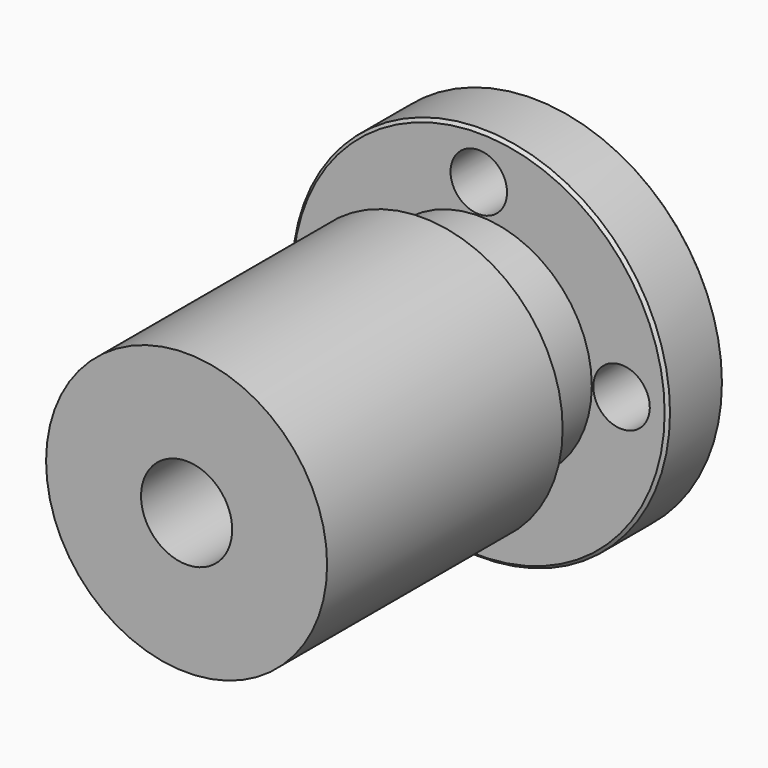
from build123d import *

# Parameters (mm, degrees)
F0_R            = 12.7
F1_DEPTH        = 4.7625
F2_R            = 7.6
F3_DEPTH        = 4.7625
F4_R            = 9.45
F4_R_2          = 7.6
F5_DEPTH        = 19.8
F6_SIZE         = 0.2
F7_R            = 1.9
F9_DEPTH        = 4.7625
F9_COPIES_COUNT = 4
F10_R           = 3.0655
F11_DEPTH       = 29.325


# Not quite as in the source:
# - a pattern or mirror of a feature is missing from the dataset's text; its kind, count and spacing are read off the source's solid


with BuildPart() as f1:
    # F0 (on Front) → F1 (new body)
    with BuildSketch(Plane.XZ):
        Circle(F0_R)
    extrude(amount=F1_DEPTH)

    # F2 (on face) → F3 (join)
    with BuildSketch(Plane.XZ.offset(4.7625)):
        Circle(F2_R)
    extrude(amount=F3_DEPTH)

    # F4 (on face) → F5 (join)
    with BuildSketch(Plane.XZ.offset(9.525)):
        Circle(F4_R)
        Circle(F4_R_2, mode=Mode.SUBTRACT)
        Circle(F4_R_2)
    extrude(amount=F5_DEPTH)

    # F6
    f6_edges = [f1.edges().sort_by_distance(p)[0] for p in [
        (-12.7, 0, 0),
        (-12.7, -4.7625, 0),
    ]]
    chamfer(f6_edges, length=F6_SIZE)

    # F7 (on face) → F9 (cut, through all)
    with BuildSketch(Plane(origin=(0, 0, 0), x_dir=(-1, 0, 0), z_dir=(0, 1, 0))):
        with Locations((0, 9.6)):
            Circle(F7_R)
    f9 = extrude(amount=-F9_DEPTH, mode=Mode.SUBTRACT)

    # F9_copies: F9 ×4 about axis
    f9_copies_axis = Axis((0, 0, 0), (0, 1, 0))
    for i in range(1, F9_COPIES_COUNT):
        add(f9.rotate(f9_copies_axis, i * 360 / F9_COPIES_COUNT), mode=Mode.SUBTRACT)

    # F10 (on face) → F11 (cut, through all)
    with BuildSketch(Plane(origin=(0, 0, 0), x_dir=(-1, 0, 0), z_dir=(0, 1, 0))):
        Circle(F10_R)
    extrude(amount=-F11_DEPTH, mode=Mode.SUBTRACT)


solid = f1.part
